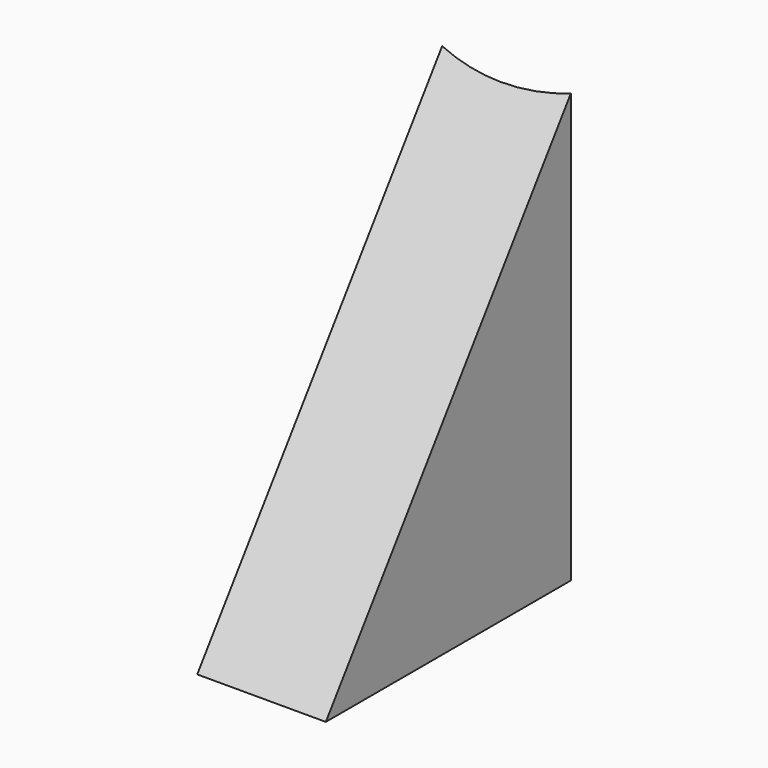
from build123d import *

# Parameters (mm, degrees)
F1_DEPTH    = 20
F2_T1_DEPTH = 109.2812333793


# Not quite as in the source:
# - a fillet or chamfer that OpenCascade refuses, or shapes differently, is made with other operations: its cross-section is extruded or revolved along the edge and cut away or added


with BuildPart() as f1:
    # F0 (on Top) → F1 (new body)
    with BuildSketch(Plane.XY):
        with BuildLine():
            Line((-3, -10), (3, -10))
            Line((3, -10), (3, 4.2837663545))
            ThreePointArc((3, 4.2837663545), (0, 4), (-3, 4.2837663545))
            Line((-3, 4.2837663545), (-3, -10))
        make_face()
    extrude(amount=F1_DEPTH)

    # F2: chamfer of 20 x 14.284 on 1 edges, made by hand

    # F2_s2 → F2_t1 (cut)
    with BuildSketch(Plane.YZ.offset(-54.6406166896)):
        Polygon((-10, 0), (4.284, 20), (-10, 20), align=None)
    extrude(amount=F2_T1_DEPTH, mode=Mode.SUBTRACT)


solid = f1.part
